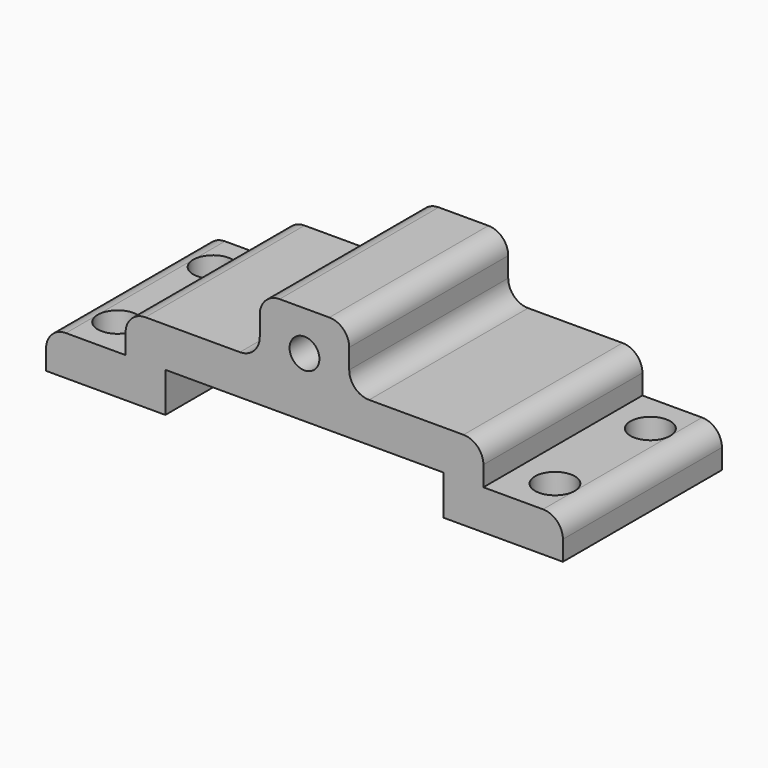
from build123d import *

# Parameters (mm, degrees)
F0_W     = 4.5
F0_H     = 3
F0_R     = 0.75
F1_DEPTH = 10
F2_R     = 1
F3_DEPTH = 4
F4_R     = 1
F5_DEPTH = 4
F6_W     = 4
F6_H     = 10
F6_R     = 1
F7_DEPTH = 2
F8_W     = 4
F8_H     = 10
F8_R     = 1
F9_DEPTH = 2
F10_R    = 0.99999


# Not quite as in the source:
# - a fillet or chamfer is up to 0.001 mm smaller than in the source, because OpenCascade refuses the exact size


with BuildPart() as f1:
    # F0 (on Front) → F1 (new body)
    with BuildSketch(Plane.XZ):
        Polygon((-13, 4), (-13, 0), (-7, 0), (-7, 2), (7, 2), (7, 0), (13, 0), (13, 4), (2.25, 4), (-2.25, 4), align=None)
        with Locations((0, 5.5)):
            Rectangle(F0_W, F0_H)
        with Locations((0, 5)):
            Circle(F0_R, mode=Mode.SUBTRACT)
    extrude(amount=F1_DEPTH)

    # F2 (on face) → F3 (cut)
    with BuildSketch(Plane.XY.offset(4)):
        with Locations((-11, -2)):
            Circle(F2_R)
        with Locations((-11, -8)):
            Circle(F2_R)
    extrude(amount=-F3_DEPTH, mode=Mode.SUBTRACT)

    # F4 (on face) → F5 (cut)
    with BuildSketch(Plane.XY.offset(4)):
        with Locations((11, -2)):
            Circle(F4_R)
        with Locations((11, -8)):
            Circle(F4_R)
    extrude(amount=-F5_DEPTH, mode=Mode.SUBTRACT)

    # F6 (on face) → F7 (cut)
    with BuildSketch(Plane.XY.offset(4)):
        with Locations((-11, -5)):
            Rectangle(F6_W, F6_H)
        with Locations((-11, -8)):
            Circle(F6_R, mode=Mode.SUBTRACT)
        with Locations((-11, -2)):
            Circle(F6_R, mode=Mode.SUBTRACT)
    extrude(amount=-F7_DEPTH, mode=Mode.SUBTRACT)

    # F8 (on face) → F9 (cut)
    with BuildSketch(Plane.XY.offset(4)):
        with Locations((11, -5)):
            Rectangle(F8_W, F8_H)
        with Locations((11, -8)):
            Circle(F8_R, mode=Mode.SUBTRACT)
        with Locations((11, -2)):
            Circle(F8_R, mode=Mode.SUBTRACT)
    extrude(amount=-F9_DEPTH, mode=Mode.SUBTRACT)

    # F10 (radius 1 in the source; OpenCascade refuses exactly that, so slightly less here)
    f10_edges = [f1.edges().sort_by_distance(p)[0] for p in [
        (-9, -5, 4),
        (-2.25, -5, 7),
        (-2.25, -5, 4),
        (2.25, -5, 7),
        (2.25, -5, 4),
        (9, -5, 4),
        (-13, -5, 2),
        (13, -5, 2),
    ]]
    fillet(f10_edges, radius=F10_R)


solid = f1.part
